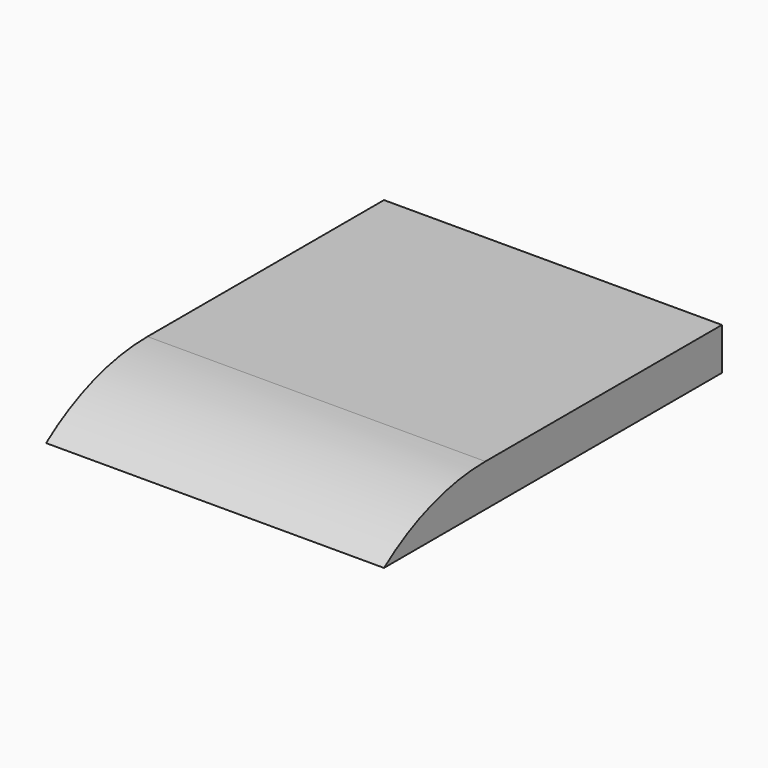
from build123d import *

# Parameters (mm, degrees)
F0_W          = 101.6
F0_H          = 12.7
F1_DEPTH      = 63.5
F1_DEPTH_BACK = 63.5
F2_T1_DEPTH   = 292.1


# Not quite as in the source:
# - a fillet or chamfer that OpenCascade refuses, or shapes differently, is made with other operations: its cross-section is extruded or revolved along the edge and cut away or added


with BuildPart() as f1:
    # F0 (on Front) → F1 (new body, two sides)
    with BuildSketch(Plane.XZ) as f1_sk:
        Rectangle(F0_W, F0_H)
    extrude(amount=F1_DEPTH)
    extrude(f1_sk.sketch, amount=-F1_DEPTH_BACK)

    # F2: fillet of radius 63.5 on 1 edges, made by hand

    # F2_s2 → F2_t1 (cut)
    with BuildSketch(Plane.YZ.offset(-146.05)):
        with BuildLine():
            ThreePointArc((-25.4, 6.35), (-45.4804631421, 3.0913894262), (-63.5, -6.35))
            Line((-63.5, -6.35), (-63.5, 6.35))
            Line((-63.5, 6.35), (-25.4, 6.35))
        make_face()
    extrude(amount=F2_T1_DEPTH, mode=Mode.SUBTRACT)


solid = f1.part
